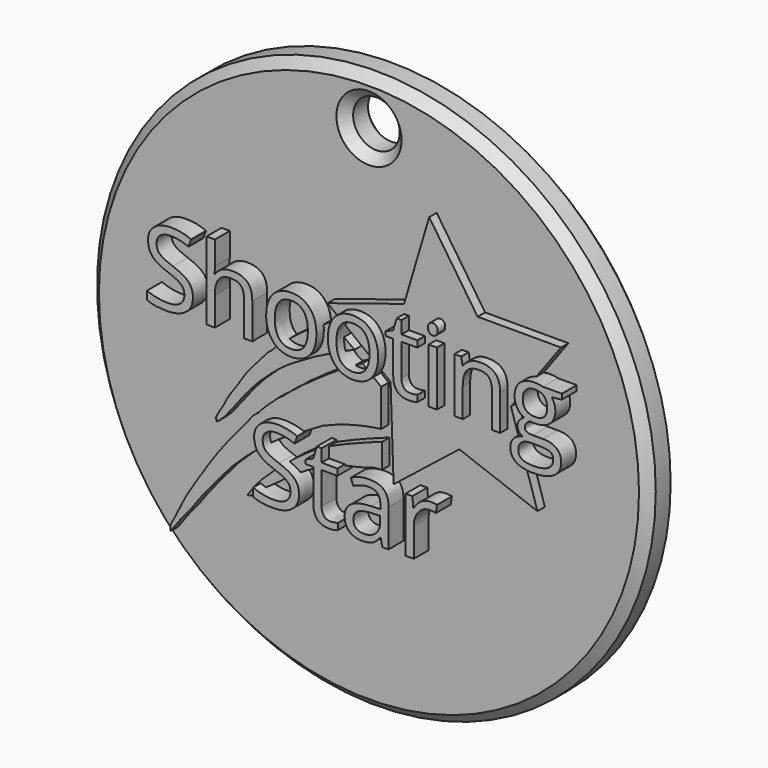
from build123d import *

# Parameters (mm, degrees)
F0_R         = 30
F0_R_2       = 2.5
F1_DEPTH     = 4
F3_START     = 2.7
F3_DEPTH     = 2.3
F4_TEXT_SIZE = 10.963675
F5_DEPTH     = 6
F6_SIZE      = 1


# Not quite as in the source:
# - Text() gives the source's letters only with a copy of the font that has no kerning and outlines rounded to 1/6400 em; it was checked with that copy


with BuildPart() as f1:
    # F0 (on Front) → F1 (new body)
    with BuildSketch(Plane.XZ):
        Circle(F0_R)
        with Locations((0, 25)):
            Circle(F0_R_2, mode=Mode.SUBTRACT)
    extrude(amount=F1_DEPTH)

    # F2 (on Front) → F3 (join)
    with BuildSketch(Plane.XZ.offset(F3_START)):
        Polygon((7.266379, 19.356208), (4.566782, 10.273928), (-3.640652, 7.674506), (3.122658, 2.427525), (3.445561, -7.143138), (10.500326, -1.541965), (18.892394, -4.662342), (16.051334, 4.308045), (21.420214, 11.632242), (12.471017, 11.632242), align=None)
        Polygon((-20.483227, -18.699549), (-20.504681, -19.361798), (-19.280439, -17.691693), (-18.330561, -16.55932), (-17.280855, -15.127316), (-16.39292, -14.035829), (-15.441673, -12.882189), (-14.682815, -11.991347), (-14.053106, -11.242504), (-13.200583, -10.413568), (-12.35775, -9.604997), (-11.339446, -8.744481), (-10.328771, -7.934637), (-8.923705, -6.921933), (-7.864262, -6.228403), (-5.799858, -5.046229), (-4.166019, -4.084647), (-2.200622, -3.302888), (-0.608188, -2.872833), (0.433361, -2.633002), (1.325285, -2.467935), (2.112421, -2.348801), (2.112421, 1.636204), (0.106754, 3.19909), (-0.465452, 2.89705), (-1.117882, 2.513068), (-1.788938, 2.137969), (-2.316669, 1.808809), (-3.022873, 1.354208), (-3.784555, 0.847539), (-4.228872, 0.536518), (-4.768922, 0.1708), (-5.707513, -0.514768), (-6.337924, -0.93961), (-7.031981, -1.516565), (-7.513157, -1.869418), (-8.048781, -2.331178), (-8.440543, -2.678798), (-9.017151, -3.067802), (-9.492542, -3.530039), (-9.914543, -3.902528), (-10.193613, -4.149398), (-10.570116, -4.534501), (-11.067517, -5.098206), (-11.574587, -5.49564), (-13.163158, -7.441987), (-14.496557, -9.074048), (-14.952832, -9.669266), (-15.356774, -10.186764), (-15.670506, -10.636744), (-16.065001, -11.197253), (-16.653458, -12.062714), (-17.019369, -12.65413), (-17.502945, -13.359434), (-17.916806, -14.024193), (-18.336551, -14.678363), (-18.856272, -15.552), (-19.304339, -16.403699), (-19.906975, -17.618529), align=None)
        Polygon((-11.396183, -12.062428), (-12.225994, -13.226188), (-12.097785, -13.261878), (-11.693928, -13.090267), (-11.337549, -12.759805), (-10.994026, -12.424153), (-10.446504, -12.042296), (-9.938421, -11.666494), (-9.170564, -11.129485), (-8.233188, -10.432039), (-7.347727, -9.843815), (-6.606597, -9.312858), (-5.707739, -8.754188), (-4.841189, -8.310346), (-3.974639, -7.850651), (-2.929223, -7.51405), (-1.81372, -7.067849), (-0.126804, -6.693499), (1.269708, -6.268474), (2.190401, -6.187517), (2.190401, -3.546653), (1.245505, -3.874742), (-0.237458, -4.439056), (-1.7232, -5.029317), (-3.301865, -5.717454), (-4.718616, -6.446068), (-5.825042, -7.181083), (-6.978682, -8.010894), (-8.340049, -9.127729), (-9.392492, -10.038498), (-10.586611, -11.171899), align=None)
        Polygon((-15.64013, -7.030844), (-15.548266, -7.372057), (-15.293485, -7.209423), (-14.975654, -6.892751), (-14.719157, -6.675364), (-14.097931, -5.88746), (-13.277513, -4.844802), (-12.809486, -4.236367), (-12.145864, -3.410742), (-11.54853, -2.74621), (-11.208147, -2.367533), (-10.557164, -1.742079), (-9.6866, -0.926616), (-8.892613, -0.269612), (-8.049555, 0.359135), (-7.344406, 0.816828), (-5.92039, 1.63775), (-4.971618, 2.200345), (-3.356571, 2.993852), (-2.001547, 3.618167), (-1.495283, 3.886505), (-0.742839, 4.216025), (-1.970885, 5.087001), (-3.264874, 6.047909), (-3.817996, 5.673488), (-4.311551, 5.362888), (-4.78975, 5.055124), (-5.433865, 4.643986), (-6.092275, 4.244116), (-6.599345, 3.863813), (-7.318836, 3.308777), (-7.941995, 2.839366), (-8.401099, 2.441932), (-8.865743, 2.060247), (-9.291222, 1.626258), (-9.64437, 1.264601), (-10.059641, 0.928915), (-10.919297, -0.066807), (-11.255425, -0.441229), (-11.710688, -0.977332), (-12.289075, -1.653875), (-12.855776, -2.503925), (-13.442716, -3.394455), (-14.029656, -4.214147), (-14.511504, -4.983568), (-14.800223, -5.587252), (-15.27267, -6.335295), align=None)
    extrude(amount=F3_DEPTH)

    # F4 (on Front) → F5 (join)
    with BuildSketch(Plane.XZ):
        with Locations((-22.796446, 2.093845)):
            Text('Shooting', F4_TEXT_SIZE, font='Open Sans', text_align=(TextAlign.LEFT, TextAlign.BOTTOM))
        with Locations((-11.401076, -12.816753)):
            Text('Star', F4_TEXT_SIZE, font='Open Sans', text_align=(TextAlign.LEFT, TextAlign.BOTTOM))
    extrude(amount=F5_DEPTH)

    # F6
    f6_edges = [f1.edges().sort_by_distance(p)[0] for p in [
        (-30, -4, 0),
        (-30, 0, 0),
        (-2.5, -4, 25),
        (-2.5, 0, 25),
    ]]
    chamfer(f6_edges, length=F6_SIZE)


solid = f1.part
